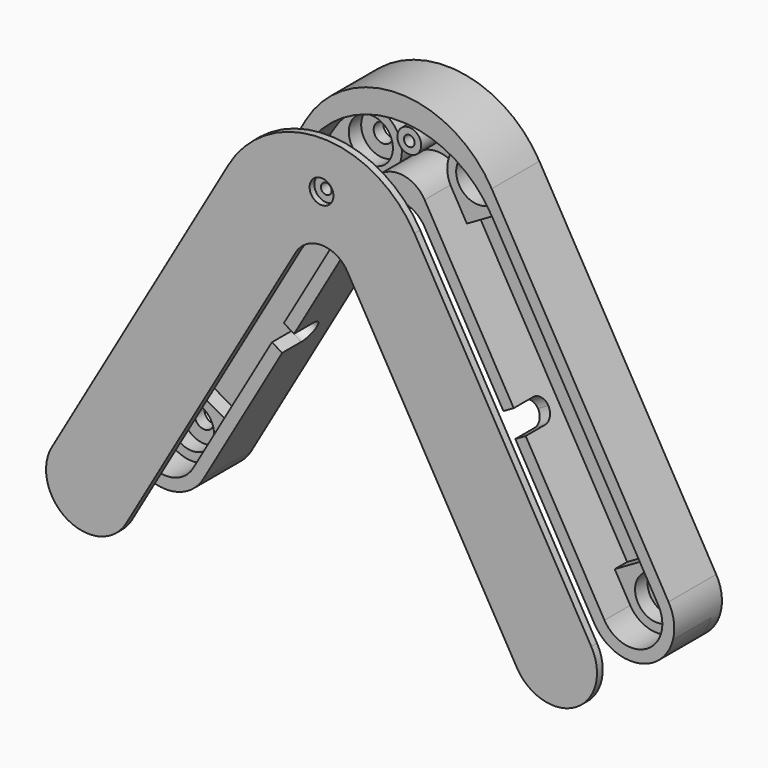
from build123d import *

# Parameters (mm, degrees)
F1_DEPTH        = 2
F3_DEPTH        = 8
F4_R            = 3.7
F5_DEPTH        = 2.6
F7_DEPTH        = 8
F9_DEPTH        = 10.001
F10_R           = 18
F11_R           = 5
F12_R           = 1.6
F13_DEPTH       = 2.001
F15_DEPTH       = 6
F16_R           = 1.99999
F17_R           = 2
F17_R_2         = 0.9
F18_DEPTH       = 5.8
F21_DEPTH       = 1.2
F23_DEPTH       = 1.2
F24_R           = 2
F25_DEPTH       = 3.4
F26_D           = 1.8
F26_CBORE_D     = 4
F26_CBORE_DEPTH = 1


# Not quite as in the source:
# - a fillet or chamfer is up to 0.001 mm smaller than in the source, because OpenCascade refuses the exact size


with BuildPart() as f1:
    # F0 (on Front) → F1 (new body)
    with BuildSketch(Plane.XZ):
        Polygon((52.5, -45.4665), (0, 45.4661673974), (-52.5, -45.4665), (-35.8723122473, -45.4665), (0, 16.6661673974), (35.8723122473, -45.4665), align=None)
    extrude(amount=F1_DEPTH)

    # F2 (on face) → F3 (join)
    with BuildSketch(Plane.XZ.offset(2)):
        Polygon((-35.8723122473, -45.4665), (0, 16.6661673974), (35.8723122473, -45.4665), (52.5, -45.4665), (0, 45.4661673974), (-52.5, -45.4665), align=None)
        Polygon((49.0358983849, -43.4665), (37.0270127857, -43.4665), (0, 20.6661673974), (-37.0270127857, -43.4665), (-49.0358983849, -43.4665), (0, 41.4661673974), align=None, mode=Mode.SUBTRACT)
    extrude(amount=F3_DEPTH)

    # F4 (on face) → F5 (join)
    with BuildSketch(Plane.XZ.offset(2)):
        with BuildLine():
            Line((-40.909996299, -29.39202473), (-43.509996299, -33.8953568297))
            ThreePointArc((-43.509996299, -33.8953568297), (-41.6066641994, -40.9986889294), (-34.5033320997, -39.0953568297))
            Line((-34.5033320997, -39.0953568297), (-31.9033320997, -34.59202473))
            Line((-31.9033320997, -34.59202473), (-40.909996299, -29.39202473))
        make_face()
        with Locations((-39.0066641994, -36.4953568297)):
            Circle(F4_R, mode=Mode.SUBTRACT)
        with BuildLine():
            Line((-7.1033320997, 8.3628352977), (-4.5033320997, 12.8661673974))
            ThreePointArc((-4.5033320997, 12.8661673974), (-6.4066641994, 19.969499497), (-13.509996299, 18.0661673974))
            Line((-13.509996299, 18.0661673974), (-16.109996299, 13.5628352977))
            Line((-16.109996299, 13.5628352977), (-7.1033320997, 8.3628352977))
        make_face()
        with Locations((-9.0066641994, 15.4661673974)):
            Circle(F4_R, mode=Mode.SUBTRACT)
        with BuildLine():
            Line((43.509996299, -33.8953568297), (40.909996299, -29.39202473))
            Line((40.909996299, -29.39202473), (31.9033320997, -34.59202473))
            Line((31.9033320997, -34.59202473), (34.5033320997, -39.0953568297))
            ThreePointArc((34.5033320997, -39.0953568297), (41.6066641994, -40.9986889294), (43.509996299, -33.8953568297))
        make_face()
        with Locations((39.0066641994, -36.4953568297)):
            Circle(F4_R, mode=Mode.SUBTRACT)
        with BuildLine():
            ThreePointArc((13.509996299, 18.0661673974), (6.4066641994, 19.969499497), (4.5033320997, 12.8661673974))
            Line((4.5033320997, 12.8661673974), (7.1033320997, 8.3628352977))
            Line((7.1033320997, 8.3628352977), (16.109996299, 13.5628352977))
            Line((16.109996299, 13.5628352977), (13.509996299, 18.0661673974))
        make_face()
        with Locations((9.0066641994, 15.4661673974)):
            Circle(F4_R, mode=Mode.SUBTRACT)
    extrude(amount=F5_DEPTH)

    # F6 (on face) → F7 (join, through all)
    with BuildSketch(Plane.XZ.offset(2)):
        with BuildLine():
            ThreePointArc((-34.5033320997, -39.0953568297), (-41.6066641994, -40.9986889294), (-43.509996299, -33.8953568297))
            Line((-43.509996299, -33.8953568297), (-45.2420471066, -32.8953568297))
            ThreePointArc((-45.2420471066, -32.8953568297), (-42.6066641994, -42.7307397369), (-32.7712812921, -40.0953568297))
            Line((-32.7712812921, -40.0953568297), (-34.5033320997, -39.0953568297))
        make_face()
        with BuildLine():
            Line((45.2420471066, -32.8953568297), (43.509996299, -33.8953568297))
            ThreePointArc((43.509996299, -33.8953568297), (41.6066641994, -40.9986889294), (34.5033320997, -39.0953568297))
            Line((34.5033320997, -39.0953568297), (32.7712812921, -40.0953568297))
            ThreePointArc((32.7712812921, -40.0953568297), (42.6066641994, -42.7307397369), (45.2420471066, -32.8953568297))
        make_face()
    extrude(amount=F7_DEPTH)

    # F8 (on face) → F9 (cut, through all)
    with BuildSketch(Plane.XZ.offset(10)):
        with BuildLine():
            ThreePointArc((-32.7712812921, -40.0953568297), (-42.6066641994, -42.7307397369), (-45.2420471066, -32.8953568297))
            Line((-45.2420471066, -32.8953568297), (-52.5, -45.4665))
            Line((-52.5, -45.4665), (-35.8723122473, -45.4665))
            Line((-35.8723122473, -45.4665), (-32.7712812921, -40.0953568297))
        make_face()
        with BuildLine():
            Line((52.5, -45.4665), (45.2420471066, -32.8953568297))
            ThreePointArc((45.2420471066, -32.8953568297), (42.6066641994, -42.7307397369), (32.7712812921, -40.0953568297))
            Line((32.7712812921, -40.0953568297), (35.8723122473, -45.4665))
            Line((35.8723122473, -45.4665), (52.5, -45.4665))
        make_face()
    extrude(amount=-F9_DEPTH, mode=Mode.SUBTRACT)

    # F10
    f10_edges = [f1.edges().sort_by_distance(p)[0] for p in [
        (0, -6, 41.466167),
        (0, -5, 45.466167),
    ]]
    fillet(f10_edges, radius=F10_R)

    # F11
    f11_edges = [f1.edges().sort_by_distance(p)[0] for p in [
        (0, -5, 16.666167),
        (0, -6, 20.666167),
    ]]
    fillet(f11_edges, radius=F11_R)

    # F12 (on face) → F13 (cut, through all)
    with BuildSketch(Plane.XZ.offset(2)):
        with Locations((-9.0066641994, 15.4661673974)):
            Circle(F12_R)
        with Locations((9.0066641994, 15.4661673974)):
            Circle(F12_R)
        with Locations((-39.0066641994, -36.4953568297)):
            Circle(F12_R)
        with Locations((39.0066641994, -36.4953568297)):
            Circle(F12_R)
    extrude(amount=-F13_DEPTH, mode=Mode.SUBTRACT)

    # F14 (on face) → F15 (cut)
    with BuildSketch(Plane.XZ.offset(10)):
        Polygon((-21.2827549631, -16.1966455237), (-19.5507041555, -17.1966455237), (-17.5507041555, -13.7325439086), (-19.2827549631, -12.7325439086), align=None)
        Polygon((19.5507041555, -17.1966455237), (21.2827549631, -16.1966455237), (19.2827549631, -12.7325439086), (17.5507041555, -13.7325439086), align=None)
    extrude(amount=-F15_DEPTH, mode=Mode.SUBTRACT)

    # F16 (radius 2 in the source; OpenCascade refuses exactly that, so slightly less here)
    f16_edges = [f1.edges().sort_by_distance(p)[0] for p in [
        (-18.41673, -4, -13.232544),
        (18.41673, -4, -13.232544),
        (20.41673, -4, -16.696646),
        (-20.41673, -4, -16.696646),
    ]]
    fillet(f16_edges, radius=F16_R)

    # F17 (on face) → F18 (join)
    with BuildSketch(Plane.XZ.offset(2)):
        with Locations((0, 19.5661673974)):
            Circle(F17_R)
        with Locations((0, 19.5661673974)):
            Circle(F17_R_2, mode=Mode.SUBTRACT)
    extrude(amount=F18_DEPTH)


with BuildPart() as f21:
    # F20 (on offset) → F21 (new body)
    with BuildSketch(Plane.XZ.offset(25)):
        with BuildLine():
            Line((45.2420471066, -32.8953568297), (15.5884572681, 18.4661673974))
            ThreePointArc((15.5884572681, 18.4661673974), (0, 27.4661673974), (-15.5884572681, 18.4661673974))
            Line((-15.5884572681, 18.4661673974), (-45.2420471066, -32.8953568297))
            ThreePointArc((-45.2420471066, -32.8953568297), (-42.6066641994, -42.7307397369), (-32.7712812921, -40.0953568297))
            Line((-32.7712812921, -40.0953568297), (-4.3301270189, 9.1661673974))
            ThreePointArc((-4.3301270189, 9.1661673974), (0, 11.6661673974), (4.3301270189, 9.1661673974))
            Line((4.3301270189, 9.1661673974), (32.7712812921, -40.0953568297))
            ThreePointArc((32.7712812921, -40.0953568297), (42.6066641994, -42.7307397369), (45.2420471066, -32.8953568297))
        make_face()
    extrude(amount=F21_DEPTH)

    # F22 (on face) → F23 (join)
    with BuildSketch(Plane(origin=(0, -25, 0), x_dir=(-1, 0, 0), z_dir=(0, 1, 0))):
        with BuildLine():
            Line((-34.5033320997, -39.0953568297), (-4.3301270189, 13.1661673974))
            ThreePointArc((-4.3301270189, 13.1661673974), (0, 15.6661673974), (4.3301270189, 13.1661673974))
            Line((4.3301270189, 13.1661673974), (34.5033320997, -39.0953568297))
            ThreePointArc((34.5033320997, -39.0953568297), (41.6066641994, -40.9986889294), (43.509996299, -33.8953568297))
            Line((43.509996299, -33.8953568297), (15.5884572681, 14.4661673974))
            ThreePointArc((15.5884572681, 14.4661673974), (0, 23.4661673974), (-15.5884572681, 14.4661673974))
            Line((-15.5884572681, 14.4661673974), (-43.509996299, -33.8953568297))
            ThreePointArc((-43.509996299, -33.8953568297), (-41.6066641994, -40.9986889294), (-34.5033320997, -39.0953568297))
        make_face()
    extrude(amount=F23_DEPTH)

    # F24 (on face) → F25 (join)
    with BuildSketch(Plane.XZ.offset(26.2)):
        with Locations((0, 19.5661673974)):
            Circle(F24_R)
    extrude(amount=-F25_DEPTH)

    # F26 (through all)
    with Locations(Plane.XZ.offset(26.2)):
        with Locations((0, 19.5661673974)):
            CounterBoreHole(F26_D / 2, F26_CBORE_D / 2, F26_CBORE_DEPTH)


solid = Compound([f1.part, f21.part])
